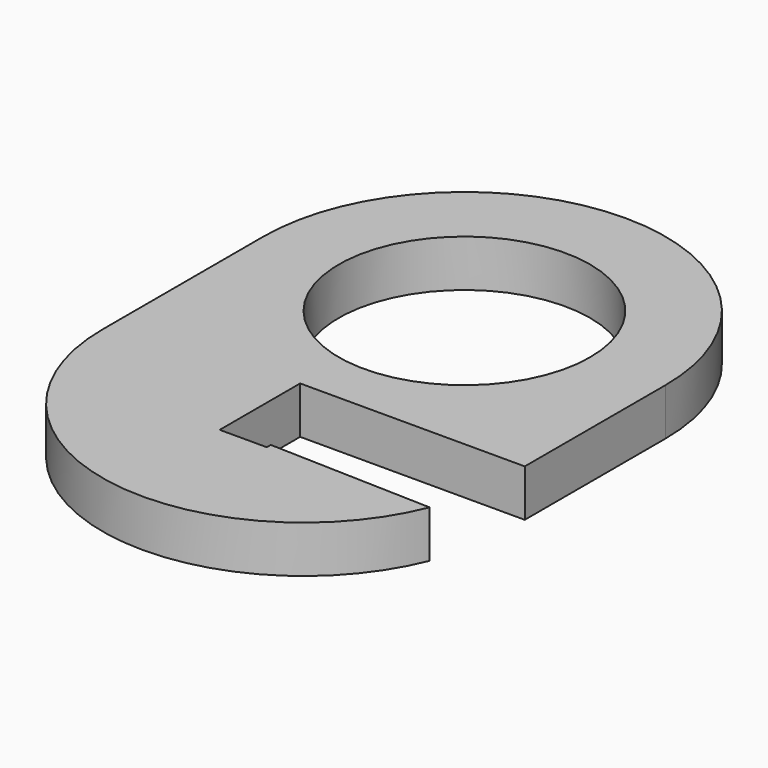
from build123d import *

# Parameters (mm, degrees)
F0_R     = 7.9375
F1_DEPTH = 2.9718
F3_DEPTH = 2.9718


# Not quite as in the source:
# - a feature names something its author has since deleted; it is built from what else it names


with BuildPart() as f1:
    # F0 (on Top) → F1 (new body)
    with BuildSketch(Plane.XY):
        with BuildLine():
            ThreePointArc((-12.7, 0), (0, -12.7), (12.7, 0))
            ThreePointArc((12.7, 0), (0, 12.7), (-12.7, 0))
        make_face()
        Circle(F0_R, mode=Mode.SUBTRACT)
        with BuildLine():
            Line((12.7, -12.7), (12.7, 0))
            ThreePointArc((12.7, 0), (0, -12.7), (-12.7, 0))
            Line((-12.7, 0), (-12.7, -12.7))
            ThreePointArc((-12.7, -12.7), (0, -25.4), (12.7, -12.7))
        make_face()
    extrude(amount=-F1_DEPTH)

    # F2 (on face) → F3 (cut, through all)
    with BuildSketch(Plane.XY):
        with BuildLine():
            Line((12.7, -11.1125), (-1.4859, -11.1125))
            Line((-1.4859, -11.1125), (-1.4859, -17.4625))
            Line((-1.4859, -17.4625), (1.4859, -17.4625))
            Line((1.4859, -17.4625), (1.4859, -17.145))
            Line((1.4859, -17.145), (11.7732150983, -17.4625))
            ThreePointArc((11.7732150983, -17.4625), (12.4661508042, -15.1259192332), (12.7, -12.7))
            Line((12.7, -12.7), (12.7, -11.1125))
        make_face()
    extrude(amount=-F3_DEPTH, mode=Mode.SUBTRACT)


solid = f1.part
